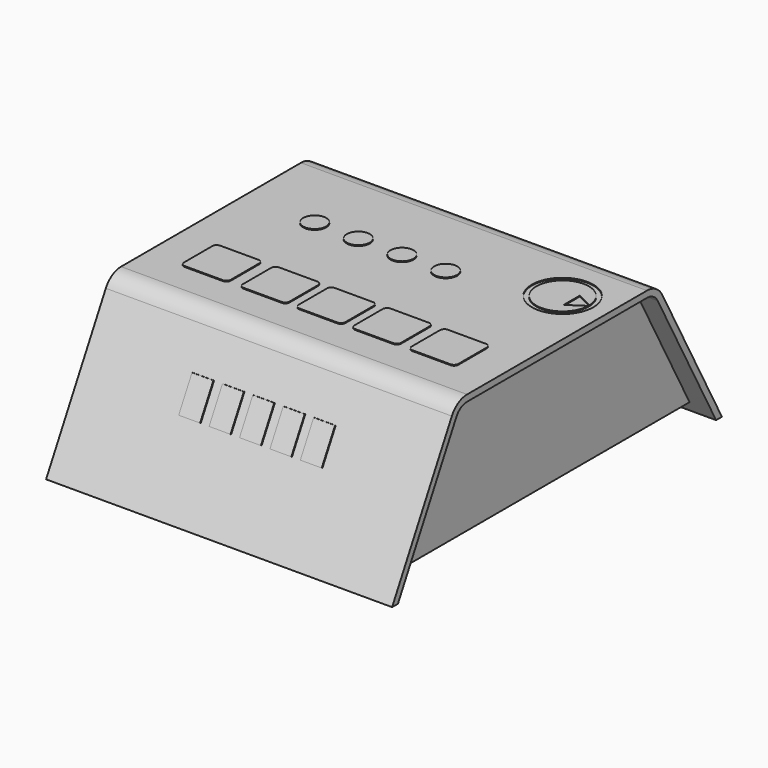
from build123d import *

# Parameters (mm, degrees)
F2_DEPTH  = 50.8
F4_W      = 6.283306625
F4_H      = 10.2798976004
F5_DEPTH  = 0.254
F7_DEPTH  = 0.254
F9_DEPTH  = 44.45
F10_R     = 3.3849263003
F11_DEPTH = 0.254
F12_R     = 9.0176977482
F13_DEPTH = 0.254


# Not quite as in the source:
# - a feature names something its author has since deleted; it is built from what else it names
# - the program builds the solid bodies; features that only make, move or delete a surface that nothing else refers to are left out


with BuildPart() as f2:
    # F1 (on Right) → F2 (new body, symmetric)
    with BuildSketch(Plane.YZ):
        with BuildLine():
            Line((-38.6035041166, 11.9795769261), (-60.5272354513, -28.4950081259))
            Line((-60.5272354513, -28.4950081259), (-58.3865008404, -28.4950081259))
            Line((-58.3865008404, -28.4950081259), (-36.9483857369, 11.0830545618))
            ThreePointArc((-36.9483857369, 11.0830545618), (-35.3062004297, 12.7935845395), (-33.02, 13.4228483819))
            Line((-33.02, 13.4228483819), (-7.4128283233, 13.4228483819))
            Line((-7.4128283233, 13.4228483819), (7.4128283233, 13.4228483819))
            Line((7.4128283233, 13.4228483819), (33.02, 13.4228483819))
            ThreePointArc((33.02, 13.4228483819), (35.3062004297, 12.7935845395), (36.9483857369, 11.0830545618))
            Line((36.9483857369, 11.0830545618), (58.3865008404, -28.4950081259))
            Line((58.3865008404, -28.4950081259), (60.5272354513, -28.4950081259))
            Line((60.5272354513, -28.4950081259), (38.6035041166, 11.9795769261))
            ThreePointArc((38.6035041166, 11.9795769261), (36.2694287388, 14.4107921406), (33.02, 15.3051791713))
            Line((33.02, 15.3051791713), (0, 15.3051791713))
            Line((0, 15.3051791713), (-33.02, 15.3051791713))
            ThreePointArc((-33.02, 15.3051791713), (-36.2694287388, 14.4107921406), (-38.6035041166, 11.9795769261))
        make_face()
    extrude(amount=F2_DEPTH, both=True)

    # F4 (on face) → F5 (join)
    with BuildSketch(Plane(origin=(0, -34.8634190503, 18.8843500603), x_dir=(1, 0, 0), z_dir=(0, -0.8792919869, 0.476283111))):
        with Locations((-17.8583269549, -24.2836587131)):
            Rectangle(F4_W, F4_H)
        with Locations((-8.9291634774, -24.2836587131)):
            Rectangle(F4_W, F4_H)
        with Locations((0, -24.2836587131)):
            Rectangle(F4_W, F4_H)
        with Locations((8.9291634774, -24.2836587131)):
            Rectangle(F4_W, F4_H)
        with Locations((17.8583269549, -24.2836587131)):
            Rectangle(F4_W, F4_H)
    extrude(amount=F5_DEPTH)

    # F6 (on face) → F7 (join)
    with BuildSketch(Plane.XY.offset(15.3051791713)):
        with BuildLine():
            Line((-28.0506481811, -11.053937773), (-39.258038976, -11.053937773))
            ThreePointArc((-39.258038976, -11.053937773), (-40.1560645881, -11.4259121609), (-40.528038976, -12.323937773))
            Line((-40.528038976, -12.323937773), (-40.528038976, -22.7773072362))
            ThreePointArc((-40.528038976, -22.7773072362), (-40.1560645881, -23.6753328483), (-39.258038976, -24.0473072362))
            Line((-39.258038976, -24.0473072362), (-28.0506481811, -24.0473072362))
            ThreePointArc((-28.0506481811, -24.0473072362), (-27.152622569, -23.6753328483), (-26.7806481811, -22.7773072362))
            Line((-26.7806481811, -22.7773072362), (-26.7806481811, -12.323937773))
            ThreePointArc((-26.7806481811, -12.323937773), (-27.152622569, -11.4259121609), (-28.0506481811, -11.053937773))
        make_face()
        with BuildLine():
            Line((-10.7684130521, -11.053937773), (-21.9758038469, -11.053937773))
            ThreePointArc((-21.9758038469, -11.053937773), (-22.873829459, -11.4259121609), (-23.2458038469, -12.323937773))
            Line((-23.2458038469, -12.323937773), (-23.2458038469, -22.7773072362))
            ThreePointArc((-23.2458038469, -22.7773072362), (-22.873829459, -23.6753328483), (-21.9758038469, -24.0473072362))
            Line((-21.9758038469, -24.0473072362), (-10.7684130521, -24.0473072362))
            ThreePointArc((-10.7684130521, -24.0473072362), (-9.87038744, -23.6753328483), (-9.4984130521, -22.7773072362))
            Line((-9.4984130521, -22.7773072362), (-9.4984130521, -12.323937773))
            ThreePointArc((-9.4984130521, -12.323937773), (-9.87038744, -11.4259121609), (-10.7684130521, -11.053937773))
        make_face()
        with BuildLine():
            Line((5.6036953974, -11.053937773), (-5.6036953974, -11.053937773))
            ThreePointArc((-5.6036953974, -11.053937773), (-6.5017210095, -11.4259121609), (-6.8736953974, -12.323937773))
            Line((-6.8736953974, -12.323937773), (-6.8736953974, -22.7773072362))
            ThreePointArc((-6.8736953974, -22.7773072362), (-6.5017210095, -23.6753328483), (-5.6036953974, -24.0473072362))
            Line((-5.6036953974, -24.0473072362), (5.6036953974, -24.0473072362))
            ThreePointArc((5.6036953974, -24.0473072362), (6.5017210095, -23.6753328483), (6.8736953974, -22.7773072362))
            Line((6.8736953974, -22.7773072362), (6.8736953974, -12.323937773))
            ThreePointArc((6.8736953974, -12.323937773), (6.5017210095, -11.4259121609), (5.6036953974, -11.053937773))
        make_face()
        with BuildLine():
            Line((21.9758038469, -11.053937773), (10.7684130521, -11.053937773))
            ThreePointArc((10.7684130521, -11.053937773), (9.87038744, -11.4259121609), (9.4984130521, -12.323937773))
            Line((9.4984130521, -12.323937773), (9.4984130521, -22.7773072362))
            ThreePointArc((9.4984130521, -22.7773072362), (9.87038744, -23.6753328483), (10.7684130521, -24.0473072362))
            Line((10.7684130521, -24.0473072362), (21.9758038469, -24.0473072362))
            ThreePointArc((21.9758038469, -24.0473072362), (22.873829459, -23.6753328483), (23.2458038469, -22.7773072362))
            Line((23.2458038469, -22.7773072362), (23.2458038469, -12.323937773))
            ThreePointArc((23.2458038469, -12.323937773), (22.873829459, -11.4259121609), (21.9758038469, -11.053937773))
        make_face()
        with BuildLine():
            Line((38.7882444791, -11.053937773), (27.5808536842, -11.053937773))
            ThreePointArc((27.5808536842, -11.053937773), (26.6828280721, -11.4259121609), (26.3108536842, -12.323937773))
            Line((26.3108536842, -12.323937773), (26.3108536842, -22.7773072362))
            ThreePointArc((26.3108536842, -22.7773072362), (26.6828280721, -23.6753328483), (27.5808536842, -24.0473072362))
            Line((27.5808536842, -24.0473072362), (38.7882444791, -24.0473072362))
            ThreePointArc((38.7882444791, -24.0473072362), (39.6862700912, -23.6753328483), (40.0582444791, -22.7773072362))
            Line((40.0582444791, -22.7773072362), (40.0582444791, -12.323937773))
            ThreePointArc((40.0582444791, -12.323937773), (39.6862700912, -11.4259121609), (38.7882444791, -11.053937773))
        make_face()
    extrude(amount=F7_DEPTH)

    # F10 (on face) → F11 (join)
    with BuildSketch(Plane.XY.offset(15.3051791713)):
        with Locations((-29.6148993075, 11.5722091869)):
            Circle(F10_R)
        with Locations((-16.793559286, 11.5722091869)):
            Circle(F10_R)
        with Locations((-3.9722192645, 11.5722091869)):
            Circle(F10_R)
        with Locations((8.849120757, 11.5722091869)):
            Circle(F10_R)
    extrude(amount=F11_DEPTH)

    # F12 (on face) → F13 (cut)
    with BuildSketch(Plane.XY.offset(15.3051791713)):
        with Locations((37.3422021844, 18.8740905886)):
            Circle(F12_R)
        with BuildLine():
            ThreePointArc((45.0367882661, 19.0583374351), (45.0384424307, 18.9662206123), (45.0389938452, 18.8740905886))
            ThreePointArc((45.0389938452, 18.8740905886), (45.0384424307, 18.781960565), (45.0367882661, 18.6898437421))
            ThreePointArc((45.0367882661, 18.6898437421), (29.6454105237, 18.8740905886), (45.0367882661, 19.0583374351))
        make_face(mode=Mode.SUBTRACT)
        with BuildLine():
            ThreePointArc((45.0367882661, 18.6898437421), (45.0384424307, 18.781960565), (45.0389938452, 18.8740905886))
            ThreePointArc((45.0389938452, 18.8740905886), (45.0384424307, 18.9662206123), (45.0367882661, 19.0583374351))
            Line((45.0367882661, 19.0583374351), (40.3160825372, 21.4442182332))
            Line((40.3160825372, 21.4442182332), (40.3160825372, 15.5540443957))
            Line((40.3160825372, 15.5540443957), (45.0367882661, 18.6898437421))
        make_face()
    extrude(amount=-F13_DEPTH, mode=Mode.SUBTRACT)


with BuildPart() as f9:
    # F8 (on Right) → F9 (new body, symmetric)
    with BuildSketch(Plane.YZ):
        with BuildLine():
            Line((-36.9483857369, 11.0830545618), (-56.5905375594, -25.1793832691))
            Line((-56.5905375594, -25.1793832691), (56.5905375594, -25.1793832691))
            Line((56.5905375594, -25.1793832691), (36.9483857369, 11.0830545618))
            ThreePointArc((36.9483857369, 11.0830545618), (35.3062004297, 12.7935845395), (33.02, 13.4228483819))
            Line((33.02, 13.4228483819), (-33.02, 13.4228483819))
            ThreePointArc((-33.02, 13.4228483819), (-35.3062004297, 12.7935845395), (-36.9483857369, 11.0830545618))
        make_face()
    extrude(amount=F9_DEPTH, both=True)


solid = Compound([f2.part, f9.part])
